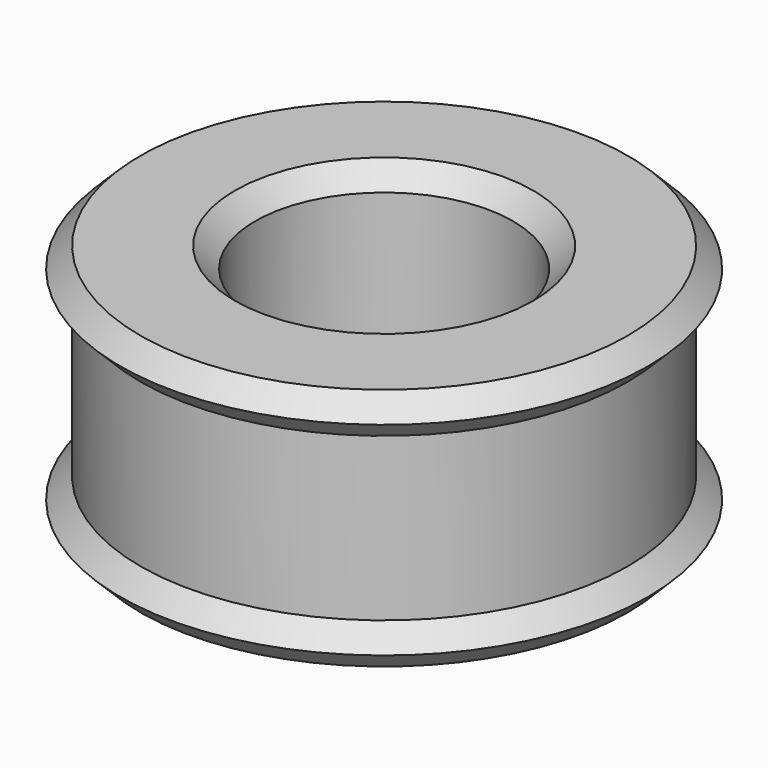
from build123d import *

# Parameters (mm, degrees)
F0_R     = 24
F0_R_2   = 12.7
F1_DEPTH = 24
F0_R_3   = 26
F2_DEPTH = 4
F3_START = 20
F3_DEPTH = 4
F4_SIZE  = 1.99999


# Not quite as in the source:
# - a fillet or chamfer is up to 0.001 mm smaller than in the source, because OpenCascade refuses the exact size


with BuildPart() as f1:
    # F0 (on Top) → F1 (new body)
    with BuildSketch(Plane.XY):
        Circle(F0_R)
        Circle(F0_R_2, mode=Mode.SUBTRACT)
    extrude(amount=F1_DEPTH)

    # F0 (on Top) → F2 (join)
    with BuildSketch(Plane.XY):
        Circle(F0_R_3)
        Circle(F0_R, mode=Mode.SUBTRACT)
    extrude(amount=F2_DEPTH)

    # F0 (on Top) → F3 (join)
    with BuildSketch(Plane.XY.offset(F3_START)):
        Circle(F0_R_3)
        Circle(F0_R, mode=Mode.SUBTRACT)
    extrude(amount=F3_DEPTH)

    # F4 (size 2 in the source; OpenCascade refuses exactly that, so slightly less here)
    f4_edges = [f1.edges().sort_by_distance(p)[0] for p in [
        (-26, 0, 20),
        (-26, 0, 24),
        (-26, 0, 4),
        (-26, 0, 0),
        (-12.7, 0, 0),
        (12.7, 0, 12),
        (-12.7, 0, 24),
    ]]
    chamfer(f4_edges, length=F4_SIZE)


solid = f1.part
